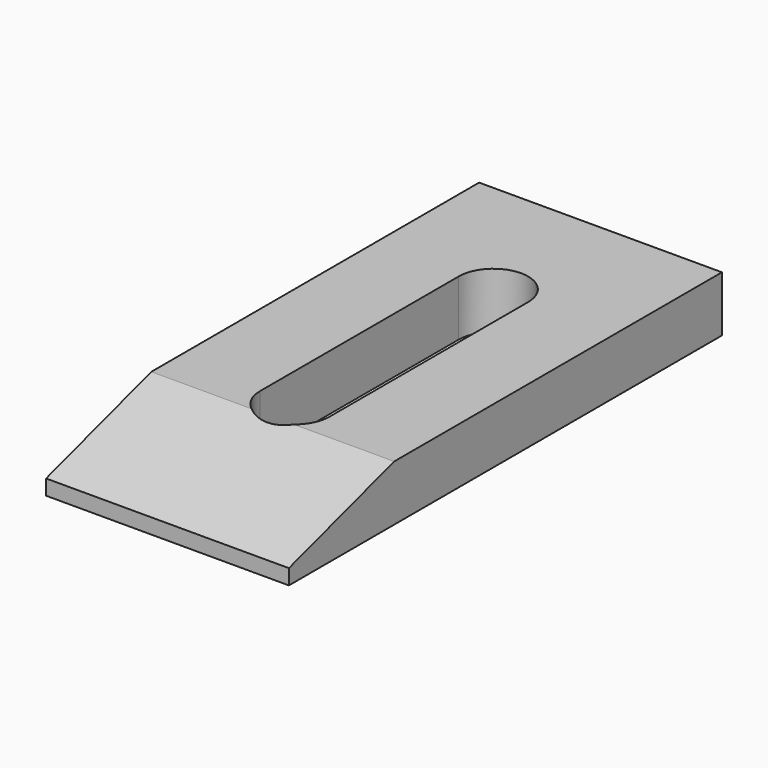
from build123d import *

# Parameters (mm, degrees)
F1_DEPTH = 24
F3_DEPTH = 11.001
F4_DEPTH = 25.8


# Not quite as in the source:
# - a feature names something its author has since deleted; it is built from what else it names


with BuildPart() as f1:
    # F0 (on Right) → F1 (new body, symmetric)
    with BuildSketch(Plane.YZ):
        Polygon((-56, 3.0059725977), (-56, 0), (51, 0), (51, 11), (-29.9936849624, 11), align=None)
    extrude(amount=F1_DEPTH, both=True)

    # F2 (on Top) → F3 (cut, through all)
    with BuildSketch(Plane.XY):
        with BuildLine():
            ThreePointArc((-6.8629677407, 24.5349109173), (0, 17.6719431765), (6.8629677407, 24.5349109173))
            Line((6.8629677407, 24.5349109173), (-6.8629677407, 24.5349109173))
        make_face()
        with BuildLine():
            Line((-6.8629677407, 24.5349109173), (6.8629677407, 24.5349109173))
            ThreePointArc((6.8629677407, 24.5349109173), (0, 31.397878658), (-6.8629677407, 24.5349109173))
        make_face()
        with BuildLine():
            Line((6.8629677407, -24.5349109173), (6.8629677407, 24.5349109173))
            ThreePointArc((6.8629677407, 24.5349109173), (0, 17.6719431765), (-6.8629677407, 24.5349109173))
            Line((-6.8629677407, 24.5349109173), (-6.8629677407, -24.5349109173))
            ThreePointArc((-6.8629677407, -24.5349109173), (0, -17.6719431765), (6.8629677407, -24.5349109173))
        make_face()
        with BuildLine():
            ThreePointArc((-6.8629677407, -24.5349109173), (0, -31.397878658), (6.8629677407, -24.5349109173))
            Line((6.8629677407, -24.5349109173), (-6.8629677407, -24.5349109173))
        make_face()
        with BuildLine():
            Line((-6.8629677407, -24.5349109173), (6.8629677407, -24.5349109173))
            ThreePointArc((6.8629677407, -24.5349109173), (0, -17.6719431765), (-6.8629677407, -24.5349109173))
        make_face()
    extrude(amount=F3_DEPTH, mode=Mode.SUBTRACT)

    # F2 (on Top) → F4 (cut)
    with BuildSketch(Plane.XY):
        with BuildLine():
            ThreePointArc((-6.8629677407, 24.5349109173), (0, 17.6719431765), (6.8629677407, 24.5349109173))
            Line((6.8629677407, 24.5349109173), (-6.8629677407, 24.5349109173))
        make_face()
        with BuildLine():
            Line((-6.8629677407, 24.5349109173), (6.8629677407, 24.5349109173))
            ThreePointArc((6.8629677407, 24.5349109173), (0, 31.397878658), (-6.8629677407, 24.5349109173))
        make_face()
        with BuildLine():
            Line((6.8629677407, -24.5349109173), (6.8629677407, 24.5349109173))
            ThreePointArc((6.8629677407, 24.5349109173), (0, 17.6719431765), (-6.8629677407, 24.5349109173))
            Line((-6.8629677407, 24.5349109173), (-6.8629677407, -24.5349109173))
            ThreePointArc((-6.8629677407, -24.5349109173), (0, -17.6719431765), (6.8629677407, -24.5349109173))
        make_face()
        with BuildLine():
            ThreePointArc((-6.8629677407, -24.5349109173), (0, -31.397878658), (6.8629677407, -24.5349109173))
            Line((6.8629677407, -24.5349109173), (-6.8629677407, -24.5349109173))
        make_face()
        with BuildLine():
            Line((-6.8629677407, -24.5349109173), (6.8629677407, -24.5349109173))
            ThreePointArc((6.8629677407, -24.5349109173), (0, -17.6719431765), (-6.8629677407, -24.5349109173))
        make_face()
    extrude(amount=F4_DEPTH, mode=Mode.SUBTRACT)


solid = f1.part
